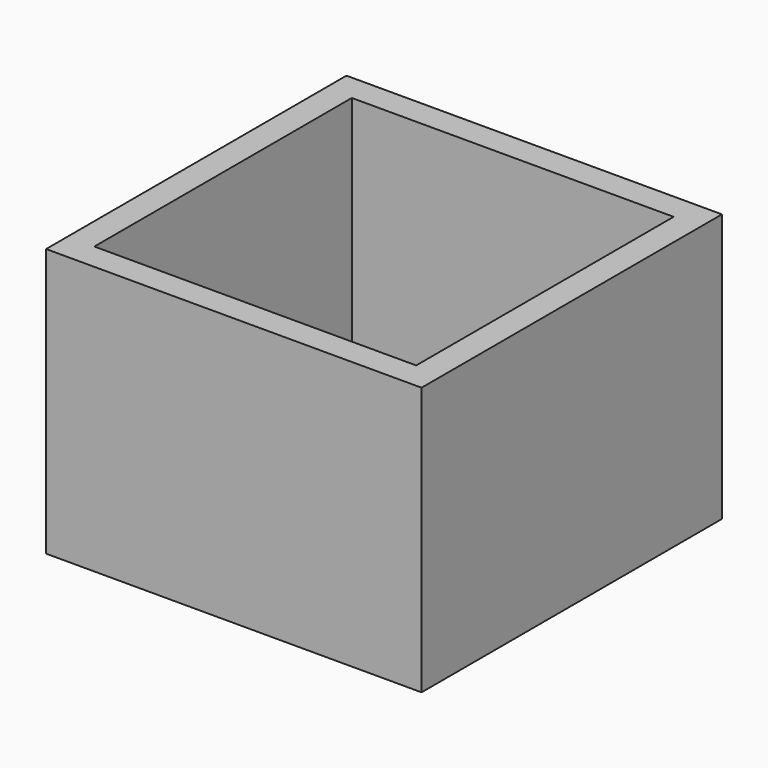
from build123d import *

# Parameters (mm, degrees)
F1_W     = 177.8
F1_H     = 177.8
F3_DEPTH = 127
F4_T     = -12.7


# Not quite as in the source:
# - a variable given as a bare number and used for a length is read in inches; the dataset says mm whatever the document's units were


with BuildPart() as f3:
    # F1 (on Top) → F3 (new body)
    with BuildSketch(Plane.XY):
        with Locations((-37.0218022674, -2.984662973)):
            Rectangle(F1_W, F1_H)
    extrude(amount=F3_DEPTH)

    # F4
    f4_openings = [f3.faces().sort_by_distance(p)[0] for p in [
        (-37.021802, -2.984663, 127),
    ]]
    offset(amount=F4_T, openings=f4_openings)


solid = f3.part
